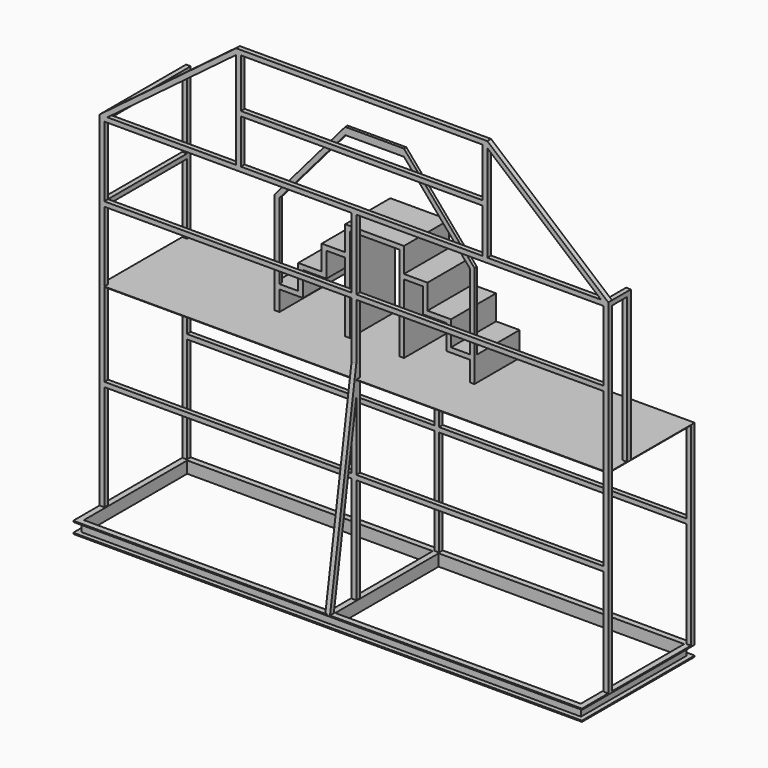
from build123d import *

# Parameters (mm, degrees)
F0_W          = 4330
F0_H          = 1200
F0_W_2        = 2090
F0_H_2        = 1100
F1_DEPTH      = 100
F2_W          = 40
F2_H          = 80
F3_DEPTH      = 4330.001
F4_W          = 40
F4_H          = 80
F5_DEPTH      = 1160.001
F7_W          = 90
F7_H          = 80
F8_DEPTH      = 550
F8_DEPTH_BACK = 550
F9_W          = 40
F9_H          = 41.1868984448
F9_H_2        = 40
F10_DEPTH     = 2930
F11_W         = 4330
F11_H         = 920
F12_DEPTH     = 4
F13_DEPTH     = 1650
F14_W         = 40
F14_H         = 40
F15_DEPTH     = 4300
F16_W         = 40
F16_H         = 40
F17_DEPTH     = 920
F19_DEPTH     = 20
F22_DEPTH     = 480
F23_W         = 2058.6071851103
F23_H         = 40
F24_DEPTH     = 40
F25_W         = 40
F25_H         = 40
F26_DEPTH     = 1250
F27_W         = 40
F27_H         = 40
F28_DEPTH     = 240
F30_DEPTH     = 25


# Not quite as in the source:
# - a feature names something its author has since deleted; it is built from what else it names


with BuildPart() as f1:
    # F0 (on Top) → F1 (new body)
    with BuildSketch(Plane.XY):
        Rectangle(F0_W, F0_H)
        with Locations((-1070, 0)):
            Rectangle(F0_W_2, F0_H_2, mode=Mode.SUBTRACT)
        with Locations((1070, 0)):
            Rectangle(F0_W_2, F0_H_2, mode=Mode.SUBTRACT)
    extrude(amount=F1_DEPTH)

    # F2 (on face) → F3 (cut, through all)
    with BuildSketch(Plane(origin=(-2165, 0, 0), x_dir=(0, -1, 0), z_dir=(-1, 0, 0))):
        with Locations((-580, 50)):
            Rectangle(F2_W, F2_H)
        with Locations((580, 50)):
            Rectangle(F2_W, F2_H)
    extrude(amount=-F3_DEPTH, mode=Mode.SUBTRACT)

    # F4 (on face) → F5 (cut, through all)
    with BuildSketch(Plane.XZ.offset(560)):
        with Locations((2145, 50)):
            Rectangle(F4_W, F4_H)
        with Locations((-2145, 50)):
            Rectangle(F4_W, F4_H)
    extrude(amount=-F5_DEPTH, mode=Mode.SUBTRACT)

    # F7 (on Front) → F8 (cut, two sides)
    with BuildSketch(Plane.XZ) as f8_sk:
        with Locations((-45, 50)):
            Rectangle(F7_W, F7_H)
    extrude(amount=-F8_DEPTH, mode=Mode.SUBTRACT)
    extrude(f8_sk.sketch, amount=F8_DEPTH_BACK, mode=Mode.SUBTRACT)

    # F9 (on face) → F10 (join)
    with BuildSketch(Plane.XY.offset(100)):
        with Locations((0, -299.4065507776)):
            Rectangle(F9_W, F9_H)
        with Locations((2145, -300)):
            Rectangle(F9_W, F9_H_2)
        with Locations((-2145, -300)):
            Rectangle(F9_W, F9_H_2)
        with Locations((-2145, 580)):
            Rectangle(F9_W, F9_H_2)
    extrude(amount=F10_DEPTH)

    # F11 (on offset) → F12 (join)
    with BuildSketch(Plane.XY.offset(1750)):
        with Locations((0, 140)):
            Rectangle(F11_W, F11_H)
    extrude(amount=F12_DEPTH)

    # F9 (on face) → F13 (join)
    with BuildSketch(Plane.XY.offset(100)):
        with Locations((-2145, 580)):
            Rectangle(F9_W, F9_H_2)
        with Locations((2145, 580)):
            Rectangle(F9_W, F9_H_2)
        with Locations((0, 580)):
            Rectangle(F9_W, F9_H_2)
        with Locations((-2145, -300)):
            Rectangle(F9_W, F9_H_2)
        with Locations((0, -299.4065507776)):
            Rectangle(F9_W, F9_H)
        with Locations((2145, -300)):
            Rectangle(F9_W, F9_H_2)
    extrude(amount=F13_DEPTH)

    # F14 (on face) → F15 (join)
    with BuildSketch(Plane(origin=(-2165, 0, 0), x_dir=(0, -1, 0), z_dir=(-1, 0, 0))):
        with Locations((300, 3010)):
            Rectangle(F14_W, F14_H)
        with Locations((-580, 1020)):
            Rectangle(F14_W, F14_H)
        with Locations((300, 1020)):
            Rectangle(F14_W, F14_H)
        with Locations((300, 2372)):
            Rectangle(F14_W, F14_H)
    extrude(amount=-F15_DEPTH)

    # F16 (on face) → F17 (join)
    with BuildSketch(Plane.XZ.offset(320)):
        with Locations((-2145, 3010)):
            Rectangle(F16_W, F16_H)
        with Locations((-2145, 2372)):
            Rectangle(F16_W, F16_H)
    extrude(amount=-F17_DEPTH)

    # F18 (on Right) → F19 (join, symmetric)
    with BuildSketch(Plane.YZ):
        Polygon((-286.3633334637, 1830.4388523102), (-316.2524058579, 1897.7677787981), (-599.6056199074, 98.6450761557), (-559.1808541492, 98.2114738751), align=None)
    extrude(amount=F19_DEPTH, both=True)

    # F21 (on offset) → F22 (join)
    with BuildSketch(Plane.XZ.offset(-600)):
        Polygon((33.9729112002, 1754), (73.9729112002, 1754), (73.9729112002, 2344), (73.9729112002, 2384), (73.9729112002, 2594), (-426.0270887998, 2594), (-426.0270887998, 2384), (-426.0270887998, 2344), (-426.0270887998, 1754), (-386.0270887998, 1754), (-386.0270887998, 2554), (33.9729112002, 2554), align=None)
        Polygon((73.9729112002, 2384), (73.9729112002, 2344), (233.9729112002, 2344), (233.9729112002, 2134), (433.9729112002, 2134), (433.9729112002, 1964), (473.9729112002, 1964), (473.9729112002, 2174), (273.9729112002, 2174), (273.9729112002, 2384), align=None)
        Polygon((-426.0270887998, 2344), (-426.0270887998, 2384), (-626.0270887998, 2384), (-626.0270887998, 2174), (-826.0270887998, 2174), (-826.0270887998, 1964), (-786.0270887998, 1964), (-786.0270887998, 2134), (-586.0270887998, 2134), (-586.0270887998, 2344), align=None)
        Polygon((473.9729112002, 1964), (433.9729112002, 1964), (433.9729112002, 1924), (633.9729112002, 1924), (633.9729112002, 1754), (673.9729112002, 1754), (673.9729112002, 1964), align=None)
        Polygon((-786.0270887998, 1964), (-826.0270887998, 1964), (-1026.0270887998, 1964), (-1026.0270887998, 1754), (-986.0270887998, 1754), (-986.0270887998, 1924), (-786.0270887998, 1924), align=None)
    extrude(amount=F22_DEPTH)

    # F23 (on face) → F24 (join)
    with BuildSketch(Plane.XZ.offset(320)):
        Polygon((-2098.4561880843, 3030), (-1003.0238811955, 3853.9479458544), (-1003.0238811955, 3904), (-2165, 3030), align=None)
        Polygon((-1003.0238811955, 3853.9479458544), (-1003.0238811955, 3030), (-963.0238811955, 3030), (-963.0238811955, 3407), (-963.0238811955, 3447), (-963.0238811955, 3864), (1095.5833039148, 3864), (1095.5833039148, 3447), (1095.5833039148, 3407), (1095.5833039148, 3030), (1135.5833039148, 3030), (1135.5833039148, 3851.5276437165), (1135.5833039148, 3904), (-1003.0238811955, 3904), align=None)
        with Locations((66.2797113596, 3427)):
            Rectangle(F23_W, F23_H)
        Polygon((2165, 3030), (1135.5833039148, 3904), (1135.5833039148, 3851.5276437165), (2103.1968882824, 3030), align=None)
    extrude(amount=-F24_DEPTH)

    # F25 (on face) → F26 (join)
    with BuildSketch(Plane.XY.offset(1754)):
        with Locations((2145, -100)):
            Rectangle(F25_W, F25_H)
    extrude(amount=F26_DEPTH)

    # F27 (on face) → F28 (join)
    with BuildSketch(Plane.XZ.offset(320)):
        with Locations((2145, 3010)):
            Rectangle(F27_W, F27_H)
    extrude(amount=-F28_DEPTH)

    # F29 (on face) → F30 (join)
    with BuildSketch(Plane.XZ.offset(-120)):
        Polygon((-1026.0270887998, 2623.4350204468), (-1026.0270887998, 1964), (-986.0270887998, 1964), (-986.0270887998, 2608.6401382994), (-426.0270887998, 3262.0944976807), (-176.0270887998, 3262.0944976807), (-176.0270887998, 3323.5646912124), (-426.0270887998, 3323.5646912124), align=None)
        Polygon((73.9729112002, 3323.5646912124), (-176.0270887998, 3323.5646912124), (-176.0270887998, 3262.0944976807), (73.9729112002, 3262.0944976807), (633.9729112002, 2608.6401382994), (633.9729112002, 1964), (673.9729112002, 1964), (673.9729112002, 2623.4350204468), align=None)
    extrude(amount=-F30_DEPTH)


solid = f1.part
